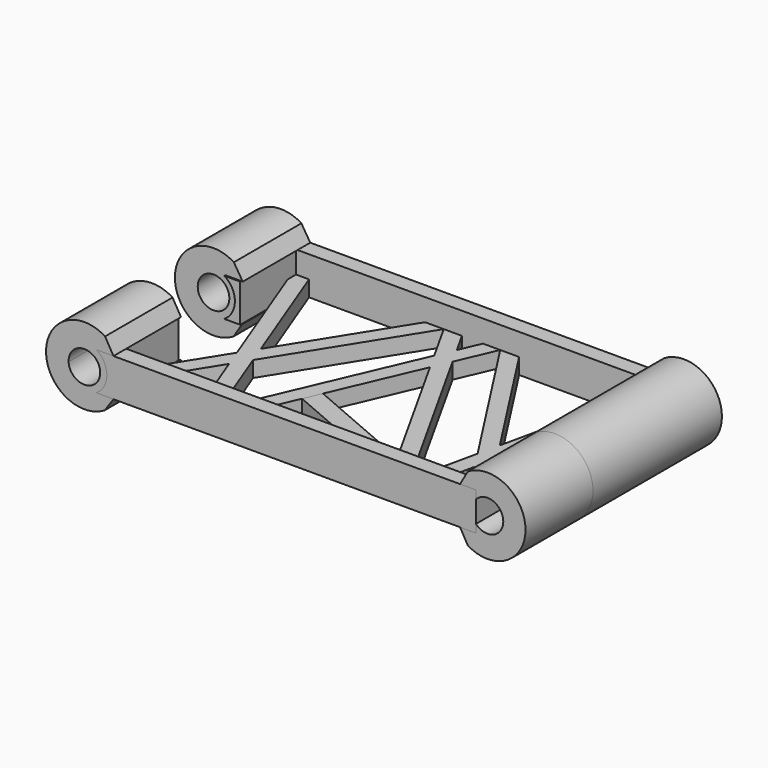
from build123d import *

# Parameters (mm, degrees)
F0_W      = 114.3
F0_H      = 73.967157311
F1_DEPTH  = 4.7752
F2_DEPTH  = 11.43
F4_D      = 13.462
F4_2_D    = 13.462
F5_R      = 4.7625
F6_DEPTH  = 25.4
F8_DEPTH  = 25.4
F9_W      = 23.2523302548
F9_H      = 11.43
F10_DEPTH = 25.4
F11_W     = 5.5641233921
F11_H     = 4.7752
F12_DEPTH = 43.434
F13_DEPTH = 48.514


# Not quite as in the source:
# - a feature names something its author has since deleted; it is built from what else it names


with BuildPart() as f1:
    # F0 (on Top) → F1 (new body)
    with BuildSketch(Plane.XY):
        with Locations((-52.6723831377, 8.9299433027)):
            Rectangle(F0_W, F0_H)
        Polygon((-105.0471831377, 37.9876717925), (-105.0471831377, 41.1383219582), (-101.1388456313, 41.1383219582), (-66.2060131753, 41.1383219582), (-60.5741511644, 41.1383219582), (-55.1043535892, 41.1383219582), (-48.7759712627, 41.1383219582), (-43.5761829824, 41.1383219582), (-37.8885207676, 41.1383219582), (-10.4127929617, 41.1383219582), (-9.5890923762, 41.1383219582), (-5.273707792, 41.1383219582), (-4.9433377569, 41.1383219582), (-0.2975831377, 41.1383219582), (-0.2975831377, 40.0308892131), (-0.2975831377, -16.9571155447), (-0.2975831377, -23.2784353529), (-1.8950043824, -23.2784353529), (-14.22920956, -23.2784353529), (-19.1186619188, -23.2784353529), (-24.5884594941, -23.2784353529), (-36.035214648, -23.2784353529), (-42.7883672511, -23.2784353529), (-71.3379746857, -23.2784353529), (-76.537762966, -23.2784353529), (-81.6493495712, -23.2784353529), (-100.8529136018, -23.2784353529), (-105.0471831377, -23.2784353529), (-105.0471831377, -20.9793318063), align=None, mode=Mode.SUBTRACT)
        Polygon((-48.5966583669, 29.4891190576), (-50.9787348492, 23.9618950121), (-24.5884594941, -23.2784353529), (-19.1186619188, -23.2784353529), align=None)
        Polygon((-50.9787348492, 23.9618950121), (-53.9140346901, 29.2162749813), (-76.537762966, -23.2784353529), (-71.3379746857, -23.2784353529), align=None)
        Polygon((-37.8885207676, 41.1383219582), (-43.5761829824, 41.1383219582), (-14.7476233332, -3.4151765974), (-13.304202216, 3.1441448502), align=None)
        Polygon((-60.5741511644, 41.1383219582), (-66.2060131753, 41.1383219582), (-87.8930449112, 6.4548268458), (-85.7575604218, 0.8631629356), align=None)
        Polygon((-4.9433377569, 41.1383219582), (-13.304202216, 3.1441448502), (-9.655600407, -2.4946375728), (-0.2975831377, 40.0308892131), (-0.2975831377, 41.1383219582), align=None)
        Polygon((-101.1388456313, 41.1383219582), (-105.0471831377, 41.1383219582), (-105.0471831377, 37.9876717925), (-91.0664245982, 1.3797248123), (-87.8930449112, 6.4548268458), align=None)
        Polygon((-91.0664245982, 1.3797248123), (-105.0471831377, -20.9793318063), (-105.0471831377, -23.2784353529), (-100.8529136018, -23.2784353529), (-88.9309401089, -4.2119390979), align=None)
        Polygon((-85.7575604218, 0.8631629356), (-88.9309401089, -4.2119390979), (-81.6493495712, -23.2784353529), (-76.537762966, -23.2784353529), align=None)
        Polygon((-9.655600407, -2.4946375728), (-11.0990215241, -9.0539590204), (-1.8950043824, -23.2784353529), (-0.2975831377, -23.2784353529), (-0.2975831377, -16.9571155447), align=None)
        Polygon((-11.0990215241, -9.0539590204), (-14.7476233332, -3.4151765974), (-19.1186619188, -23.2784353529), (-14.22920956, -23.2784353529), align=None)
        Polygon((-55.1043535892, 41.1383219582), (-60.5741511644, 41.1383219582), (-53.9140346901, 29.2162749813), (-51.5319582079, 34.7434990268), align=None)
        Polygon((-43.5761829824, 41.1383219582), (-48.7759712627, 41.1383219582), (-51.5319582079, 34.7434990268), (-48.5966583669, 29.4891190576), align=None)
        Polygon((-13.304202216, 3.1441448502), (-14.7476233332, -3.4151765974), (-11.0990215241, -9.0539590204), (-9.655600407, -2.4946375728), align=None)
        Polygon((-51.5319582079, 34.7434990268), (-53.9140346901, 29.2162749813), (-50.9787348492, 23.9618950121), (-48.5966583669, 29.4891190576), align=None)
        Polygon((-87.8930449112, 6.4548268458), (-91.0664245982, 1.3797248123), (-88.9309401089, -4.2119390979), (-85.7575604218, 0.8631629356), align=None)
    extrude(amount=F1_DEPTH)

    # F4 (through all)
    with Locations(Plane.XZ.offset(28.0536353529)):
        with Locations((-113.3868669575, 5.715)):
            Hole(F4_D / 2)


with BuildPart() as f2:
    # F0 (on Top) → F2 (new body)
    with BuildSketch(Plane.XY):
        with Locations((-52.6723831377, 8.9299433027)):
            Rectangle(F0_W, F0_H)
        Polygon((-105.0471831377, 37.9876717925), (-105.0471831377, 41.1383219582), (-101.1388456313, 41.1383219582), (-66.2060131753, 41.1383219582), (-60.5741511644, 41.1383219582), (-55.1043535892, 41.1383219582), (-48.7759712627, 41.1383219582), (-43.5761829824, 41.1383219582), (-37.8885207676, 41.1383219582), (-10.4127929617, 41.1383219582), (-9.5890923762, 41.1383219582), (-5.273707792, 41.1383219582), (-4.9433377569, 41.1383219582), (-0.2975831377, 41.1383219582), (-0.2975831377, 40.0308892131), (-0.2975831377, -16.9571155447), (-0.2975831377, -23.2784353529), (-1.8950043824, -23.2784353529), (-14.22920956, -23.2784353529), (-19.1186619188, -23.2784353529), (-24.5884594941, -23.2784353529), (-36.035214648, -23.2784353529), (-42.7883672511, -23.2784353529), (-71.3379746857, -23.2784353529), (-76.537762966, -23.2784353529), (-81.6493495712, -23.2784353529), (-100.8529136018, -23.2784353529), (-105.0471831377, -23.2784353529), (-105.0471831377, -20.9793318063), align=None, mode=Mode.SUBTRACT)
    extrude(amount=F2_DEPTH)

    # F4#2 (through all)
    with Locations(Plane.XZ.offset(28.0536353529)):
        with Locations((-113.3868669575, 5.715)):
            Hole(F4_2_D / 2)


with BuildPart() as f6:
    # F5 (on face) → F6 (new body)
    with BuildSketch(Plane(origin=(0, 45.9135219582, 0), x_dir=(-1, 0, 0), z_dir=(0, 1, 0))):
        with BuildLine():
            Line((104.8336997628, 0), (107.3452308774, -3.989065066))
            ThreePointArc((107.3452308774, -3.989065066), (125.0266367946, 5.9274575081), (107.264213264, 15.698119998))
            Line((107.264213264, 15.698119998), (104.5906469226, 11.43))
            Line((104.5906469226, 11.43), (109.8223831377, 11.43))
            Line((109.8223831377, 11.43), (109.8223831377, 11.4247124357))
            ThreePointArc((109.8223831377, 11.4247124357), (106.6558669575, 5.715), (109.8223831377, 0.0052875643))
            Line((109.8223831377, 0.0052875643), (109.8223831377, 0))
            Line((109.8223831377, 0), (104.8336997628, 0))
        make_face()
        with Locations((113.3868669575, 5.715)):
            Circle(F5_R, mode=Mode.SUBTRACT)
    extrude(amount=-F6_DEPTH)


with BuildPart() as f8:
    # F7 (on face) → F8 (new body)
    with BuildSketch(Plane.XZ.offset(28.0536353529)):
        with BuildLine():
            Line((-0.3069167142, 0), (2.00510988, -4.0852471483))
            ThreePointArc((2.00510988, -4.0852471483), (19.3918963109, 5.715), (2.00510988, 15.5152471483))
            Line((2.00510988, 15.5152471483), (-0.3069167142, 11.43))
            Line((-0.3069167142, 11.43), (4.4776168623, 11.43))
            Line((4.4776168623, 11.43), (4.4776168623, 8.9887683501))
            ThreePointArc((4.4776168623, 8.9887683501), (9.6983834917, 10.139608436), (12.6989963109, 5.715))
            ThreePointArc((12.6989963109, 5.715), (9.6983834917, 1.290391564), (4.4776168623, 2.4412316499))
            Line((4.4776168623, 2.4412316499), (4.4776168623, 0))
            Line((4.4776168623, 0), (-0.3069167142, 0))
        make_face()
    extrude(amount=-F8_DEPTH)


with BuildPart() as f8b:
    # F7 (on face) → F8, piece 2 (new body)
    with BuildSketch(Plane.XZ.offset(28.0536353529)):
        with BuildLine():
            Line((-107.2588041425, -3.7761165295), (-104.6486571431, 0))
            Line((-104.6486571431, 0), (-109.8223831377, 0))
            Line((-109.8223831377, 0), (-109.8223831377, 0.0052875643))
            ThreePointArc((-109.8223831377, 0.0052875643), (-106.6558669575, 5.715), (-109.8223831377, 11.4247124357))
            Line((-109.8223831377, 11.4247124357), (-109.8223831377, 11.43))
            Line((-109.8223831377, 11.43), (-104.6486571431, 11.43))
            Line((-104.6486571431, 11.43), (-107.1966588497, 15.7999712974))
            ThreePointArc((-107.1966588497, 15.7999712974), (-124.9681860406, 6.0682453649), (-107.2588041425, -3.7761165295))
        make_face()
        with BuildLine():
            ThreePointArc((-118.1711778045, 5.4841274396), (-113.6857560931, 10.451134302), (-108.6601093411, 6.0315144287))
            ThreePointArc((-108.6601093411, 6.0315144287), (-113.1414265767, 0.9931906529), (-118.1711778045, 5.4841274396))
        make_face(mode=Mode.SUBTRACT)
    extrude(amount=-F8_DEPTH)


with BuildPart() as f10_tool:
    # F9 (on face) → F10 (new body)
    with BuildSketch(Plane.YZ.offset(-105.0471831377)):
        with Locations((8.5088948254, 5.715)):
            Rectangle(F9_W, F9_H)
    extrude(amount=-F10_DEPTH)


with BuildPart() as f1_1:
    add(f1.part)

    # F10: cut by f10_tool
    add(f10_tool.part, mode=Mode.SUBTRACT)


with BuildPart() as f2_1:
    add(f2.part)

    # F10: cut by f10_tool
    add(f10_tool.part, mode=Mode.SUBTRACT)


with BuildPart() as f8b_1:
    add(f8b.part)

    # F10: cut by f10_tool
    add(f10_tool.part, mode=Mode.SUBTRACT)


with BuildPart() as f12:
    # F11 (on face) → F12 (new body)
    with BuildSketch(Plane(origin=(-51.702575109, 22.2823405061, 0), x_dir=(0.3957806318, 0.918345083, 0), z_dir=(0.918345083, -0.3957806318, 0))):
        with Locations((-29.4585749507, 2.3876)):
            Rectangle(F11_W, F11_H)
    extrude(amount=F12_DEPTH)


with BuildPart() as f13:
    # F13 (new): a face of the model
    f13_faces = [f8.part.faces().sort_by_distance(p)[0] for p in [
        (2.085350074, -2.6536353529, -0.3021502923),
    ]]
    extrude(f13_faces, amount=F13_DEPTH)


solid = Compound([f6.part, f8.part, f1_1.part, f2_1.part, f8b_1.part, f12.part, f13.part])
